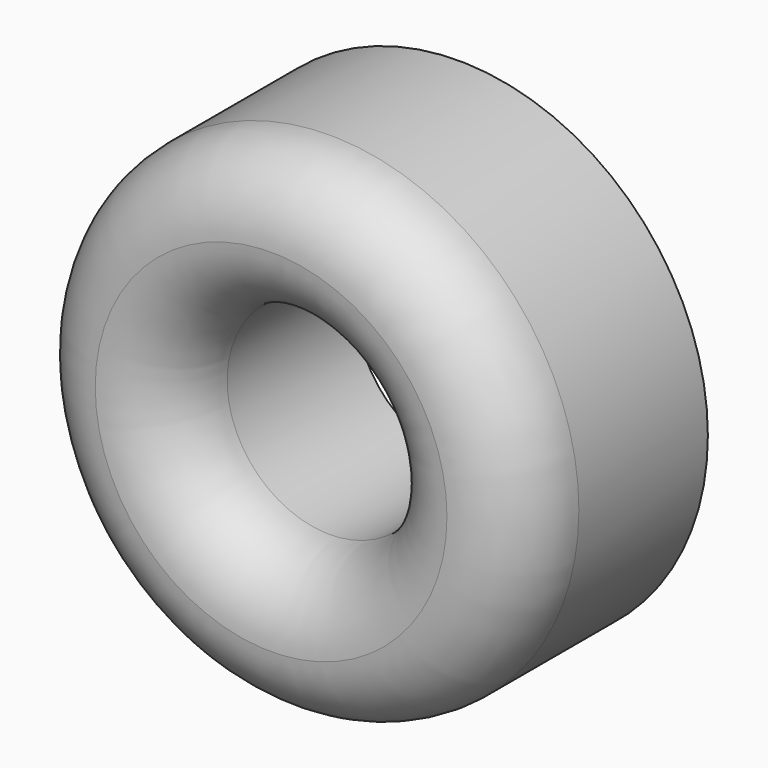
from build123d import *

# Parameters (mm, degrees)
F0_R     = 8.5
F0_R_2   = 3.5
F1_DEPTH = 8
F2_R     = 2.5
F3_R     = 2.49999


# Not quite as in the source:
# - a fillet or chamfer is up to 0.001 mm smaller than in the source, because OpenCascade refuses the exact size


with BuildPart() as f1:
    # F0 (on Front) → F1 (new body)
    with BuildSketch(Plane.XZ):
        Circle(F0_R)
        Circle(F0_R_2, mode=Mode.SUBTRACT)
    extrude(amount=F1_DEPTH)

    # F2
    f2_edges = [f1.edges().sort_by_distance(p)[0] for p in [
        (-8.5, -8, 0),
    ]]
    fillet(f2_edges, radius=F2_R)

    # F3 (radius 2.5 in the source; OpenCascade refuses exactly that, so slightly less here)
    f3_edges = [f1.edges().sort_by_distance(p)[0] for p in [
        (-3.5, -8, 0),
    ]]
    fillet(f3_edges, radius=F3_R)


solid = f1.part
